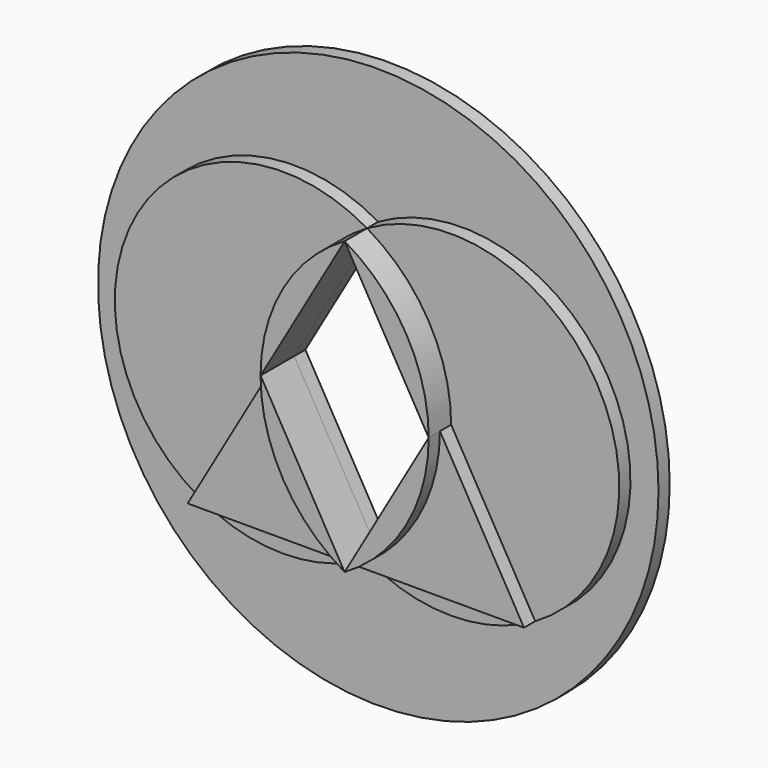
from build123d import *

# Parameters (mm, degrees)
F0_R     = 500
F2_DEPTH = 25
F3_DEPTH = 25
F4_DEPTH = 50
F5_DEPTH = 75
F6_DEPTH = 300


with BuildPart() as f2:
    # F0 (on Front) → F2 (new body)
    with BuildSketch(Plane.XZ):
        Circle(F0_R)
    extrude(amount=-F2_DEPTH)

    # F1 (on Front) → F6 (cut)
    with BuildSketch(Plane.XZ):
        Polygon((0, 0), (0, 259.8076211353), (-150, 0), align=None)
        Polygon((0, 0), (150, 0), (0, 259.8076211353), align=None)
        Polygon((0, -259.8076211353), (150, 0), (0, 0), align=None)
        Polygon((-150, 0), (0, -259.8076211353), (0, 0), align=None)
    extrude(amount=-F6_DEPTH, mode=Mode.SUBTRACT)


with BuildPart() as f3:
    # F1 (on Front) → F3 (new body)
    with BuildSketch(Plane.XZ):
        with BuildLine():
            ThreePointArc((0, 259.8076211353), (109.8076211353, 150), (150, 0))
            Line((150, 0), (300, -259.8076211353))
            ThreePointArc((300, -259.8076211353), (409.8076211353, -150), (450, 0))
            ThreePointArc((450, 0), (300, 259.8076211353), (0, 259.8076211353))
        make_face()
    extrude(amount=F3_DEPTH)


with BuildPart() as f3b:
    # F1 (on Front) → F3, piece 2 (new body)
    with BuildSketch(Plane.XZ):
        with BuildLine():
            ThreePointArc((-150, 0), (-109.8076211353, 150), (0, 259.8076211353))
            ThreePointArc((0, 259.8076211353), (-409.8076211353, 150), (-300, -259.8076211353))
            Line((-300, -259.8076211353), (-150, 0))
        make_face()
    extrude(amount=F3_DEPTH)


with BuildPart() as f3c:
    # F1 (on Front) → F3, piece 3 (new body)
    with BuildSketch(Plane.XZ):
        with BuildLine():
            Line((300, -259.8076211353), (0, -259.8076211353))
            ThreePointArc((0, -259.8076211353), (150, -300), (300, -259.8076211353))
        make_face()
    extrude(amount=F3_DEPTH)


with BuildPart() as f3d:
    # F1 (on Front) → F3, piece 4 (new body)
    with BuildSketch(Plane.XZ):
        with BuildLine():
            ThreePointArc((-300, -259.8076211353), (-150, -300), (0, -259.8076211353))
            Line((0, -259.8076211353), (-300, -259.8076211353))
        make_face()
    extrude(amount=F3_DEPTH)


with BuildPart() as f4:
    # F1 (on Front) → F4 (new body)
    with BuildSketch(Plane.XZ):
        with BuildLine():
            Line((300, -259.8076211353), (150, 0))
            ThreePointArc((150, 0), (109.8076211353, -150), (0, -259.8076211353))
            Line((0, -259.8076211353), (300, -259.8076211353))
        make_face()
    extrude(amount=F4_DEPTH)


with BuildPart() as f4b:
    # F1 (on Front) → F4, piece 2 (new body)
    with BuildSketch(Plane.XZ):
        with BuildLine():
            Line((-150, 0), (0, 259.8076211353))
            ThreePointArc((0, 259.8076211353), (-109.8076211353, 150), (-150, 0))
        make_face()
    extrude(amount=F4_DEPTH)

    # F1 (on Front) → F5, piece 3 (join)
    with BuildSketch(Plane.XZ):
        with BuildLine():
            Line((-150, 0), (0, 259.8076211353))
            ThreePointArc((0, 259.8076211353), (-109.8076211353, 150), (-150, 0))
        make_face()
    extrude(amount=F5_DEPTH)


with BuildPart() as f4c:
    # F1 (on Front) → F4, piece 3 (new body)
    with BuildSketch(Plane.XZ):
        with BuildLine():
            Line((-300, -259.8076211353), (0, -259.8076211353))
            ThreePointArc((0, -259.8076211353), (-109.8076211353, -150), (-150, 0))
            Line((-150, 0), (-300, -259.8076211353))
        make_face()
    extrude(amount=F4_DEPTH)


with BuildPart() as f5:
    # F1 (on Front) → F5 (new body)
    with BuildSketch(Plane.XZ):
        with BuildLine():
            Line((0, 259.8076211353), (150, 0))
            ThreePointArc((150, 0), (109.8076211353, 150), (0, 259.8076211353))
        make_face()
    extrude(amount=F5_DEPTH)


with BuildPart() as f5b:
    # F1 (on Front) → F5, piece 2 (new body)
    with BuildSketch(Plane.XZ):
        with BuildLine():
            ThreePointArc((0, -259.8076211353), (109.8076211353, -150), (150, 0))
            Line((150, 0), (0, -259.8076211353))
        make_face()
    extrude(amount=F5_DEPTH)


with BuildPart() as f5c:
    # F1 (on Front) → F5, piece 4 (new body)
    with BuildSketch(Plane.XZ):
        with BuildLine():
            ThreePointArc((-150, 0), (-109.8076211353, -150), (0, -259.8076211353))
            Line((0, -259.8076211353), (-150, 0))
        make_face()
    extrude(amount=F5_DEPTH)


solid = Compound([f2.part, f3.part, f3b.part, f3c.part, f3d.part, f4.part, f4b.part, f4c.part, f5.part, f5b.part, f5c.part])
